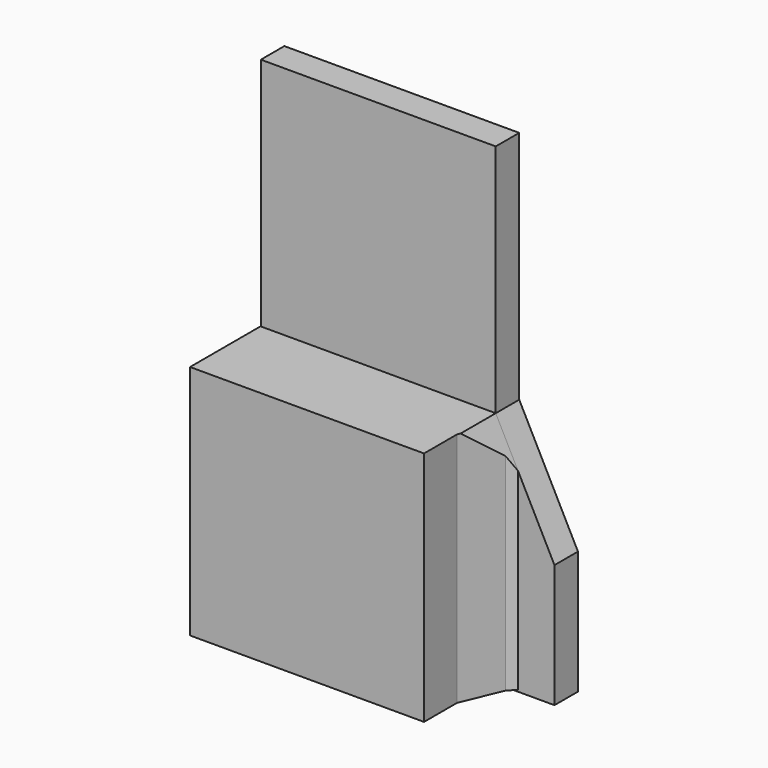
from build123d import *

# Parameters (mm, degrees)
F0_W        = 50.8
F0_H        = 26.0105735242
F1_DEPTH    = 6.35
F2_W        = 50.6046172231
F2_H        = 51.1175021529
F3_DEPTH    = 25.4
F4_T4_DEPTH = 51.1175021529
F4_T9_DEPTH = 64.038633205
F5_SIZE     = 5.08


# Not quite as in the source:
# - a fillet or chamfer that OpenCascade refuses, or shapes differently, is made with other operations: its cross-section is extruded or revolved along the edge and cut away or added


with BuildPart() as f1:
    # F0 (on Front) → F1 (new body)
    with BuildSketch(Plane.XZ):
        with Locations((0, -37.7947132379)):
            Rectangle(F0_W, F0_H)
        Polygon((-38.1, -24.7894264758), (-25.4, -24.7894264758), (-25.4, 0), align=None)
        Polygon((25.4, -50.8), (-25.4, -50.8), (-25.4, -24.7894264758), (-38.1, -24.7894264758), (-38.1, -51.4594204724), (38.1, -51.4594204724), (38.1, -24.7894264758), (25.4, -24.7894264758), align=None)
        Polygon((25.4, 0), (25.4, -24.7894264758), (38.1, -24.7894264758), align=None)
        Polygon((-25.4, 0), (-25.4, -24.7894264758), (25.4, -24.7894264758), (25.4, 0), (25.4, 50.8), (-25.4, 50.8), align=None)
    extrude(amount=F1_DEPTH)

    # F2 (on Front) → F3 (join)
    with BuildSketch(Plane.XZ):
        with Locations((-0.1709619537, -25.5587510765)):
            Rectangle(F2_W, F2_H)
    extrude(amount=F3_DEPTH)

    # F4: chamfer of 5.08 on 2 edges, made by hand


with BuildPart() as f4_tool2:
    # F4_s3 → F4_t4 (new body)
    with BuildSketch(Plane.XY):
        Polygon((30.2113466579, -6.35), (25.1313466579, -11.43), (25.1313466579, -6.35), align=None)
    extrude(amount=-F4_T4_DEPTH)

    split(bisect_by=Plane(origin=(20.1193399264, 0, 10.3074436722), x_dir=(0, 1, 0), z_dir=(-0.8899999984, 0, -0.4559605278)), keep=Keep.TOP)


with BuildPart() as f1_1:
    add(f1.part)

    # F4_t1: union F4_tool2
    add(f4_tool2.part)


with BuildPart() as f4_tool7:
    # F4_s8 → F4_t9 (new body)
    with BuildSketch(Plane.XY.offset(-51.1175021529)):
        Polygon((-25.4732705653, -11.43), (-30.5532705653, -6.35), (-25.4732705653, -6.35), align=None)
    extrude(amount=F4_T9_DEPTH)

    split(bisect_by=Plane(origin=(-20.1193399264, 0, 10.3074436722), x_dir=(0, 1, 0), z_dir=(0.8899999984, 0, -0.4559605278)), keep=Keep.TOP)


with BuildPart() as f1_2:
    add(f1_1.part)

    # F4_t6: union F4_tool7
    add(f4_tool7.part)

    # F5
    f5_edges = [f1_2.edges().sort_by_distance(p)[0] for p in [
        (25.131347, -11.43, -25.558751),
        (-25.473271, -11.43, -25.63026),
    ]]
    chamfer(f5_edges, length=F5_SIZE)


solid = f1_2.part
